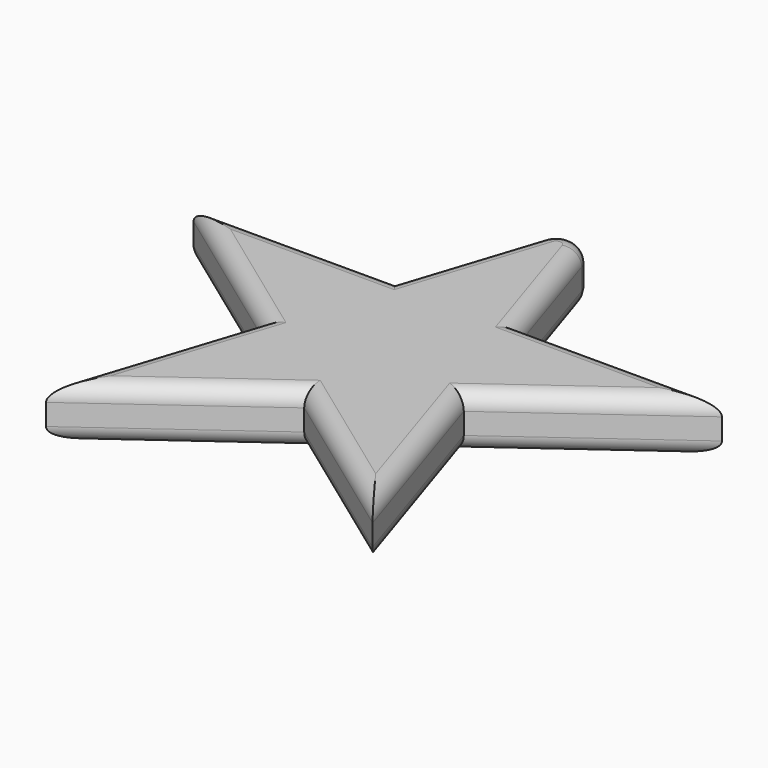
from build123d import *

# Parameters (mm, degrees)
F1_DEPTH    = 6.4
F5_R        = 1.9313708499
F6_T1_DEPTH = 6.4
F6_T4_ANGLE = 144
F6_T6_ANGLE = 144


# Not quite as in the source:
# - a fillet or chamfer that OpenCascade refuses, or shapes differently, is made with other operations: its cross-section is extruded or revolved along the edge and cut away or added


with BuildPart() as f1:
    # F0 (on Top) → F1 (new body)
    with BuildSketch(Plane.XY):
        Polygon((-31.5438667271, -25.7632551613), (-12.0486849532, -39.9273338113), (-19.495181774, -62.8452944863), (0, -48.6812158363), (19.495181774, -62.8452944863), (12.0486849532, -39.9273338113), (31.5438667271, -25.7632551613), (7.4464968208, -25.7632551613), (0, -2.8452944863), (-7.4464968208, -25.7632551613), align=None)
    extrude(amount=F1_DEPTH)

    # F5
    f5_edges = [f1.edges().sort_by_distance(p)[0] for p in [
        (-21.796276, -32.845294, 6.4),
        (-15.771933, -51.386314, 6.4),
        (-9.747591, -55.763255, 6.4),
        (9.747591, -55.763255, 6.4),
        (15.771933, -51.386314, 6.4),
        (21.796276, -32.845294, 6.4),
        (19.495182, -25.763255, 6.4),
        (3.723248, -14.304275, 6.4),
        (-3.723248, -14.304275, 6.4),
        (-19.495182, -25.763255, 6.4),
        (-21.796276, -32.845294, 0),
        (-15.771933, -51.386314, 0),
        (-9.747591, -55.763255, 0),
        (9.747591, -55.763255, 0),
        (15.771933, -51.386314, 0),
        (21.796276, -32.845294, 0),
        (19.495182, -25.763255, 0),
        (3.723248, -14.304275, 0),
        (-3.723248, -14.304275, 0),
        (-19.495182, -25.763255, 0),
    ]]
    fillet(f5_edges, radius=F5_R)

    # F6: fillet of radius 2.5491174943 on 1 edges, made by hand

    # F6_s2 → F6_t1 (cut)
    with BuildSketch(Plane.XY):
        with BuildLine():
            ThreePointArc((2.4243548038, -10.3066913542), (0, -8.5452944863), (-2.4243548038, -10.3066913542))
            Line((-2.4243548038, -10.3066913542), (0, -2.8452944863))
            Line((0, -2.8452944863), (2.4243548038, -10.3066913542))
        make_face()
    extrude(amount=F6_T1_DEPTH, mode=Mode.SUBTRACT)

    # F6_s3 → F6_t4 (revolve, cut)
    with BuildSketch(Plane(origin=(-3.2605658725, -10.0349899078, 0), x_dir=(0, 0, 1), z_dir=(-0.3090169944, -0.9510565163, 0))):
        with BuildLine():
            ThreePointArc((0, -2.8106152002), (0.5656854249, -1.4449297752), (1.9313708499, -0.8792443503))
            Line((1.9313708499, -0.8792443503), (0, -0.8792443503))
            Line((0, -0.8792443503), (0, -2.8106152002))
        make_face()
    revolve(axis=Axis((0, -11.0944119806, 0), (0, 0, -1)), revolution_arc=F6_T4_ANGLE, mode=Mode.SUBTRACT)

    # F6_s5 → F6_t6 (revolve, cut)
    with BuildSketch(Plane(origin=(3.2605658725, -10.0349899078, 0), x_dir=(0, 0, 1), z_dir=(0.3090169944, -0.9510565163, 0))):
        with BuildLine():
            ThreePointArc((6.4, 2.8106152002), (5.8343145751, 1.4449297752), (4.4686291501, 0.8792443503))
            Line((4.4686291501, 0.8792443503), (6.4, 0.8792443503))
            Line((6.4, 0.8792443503), (6.4, 2.8106152002))
        make_face()
    revolve(axis=Axis((0, -11.0944119806, 6.4), (0, 0, 1)), revolution_arc=F6_T6_ANGLE, mode=Mode.SUBTRACT)


solid = f1.part
